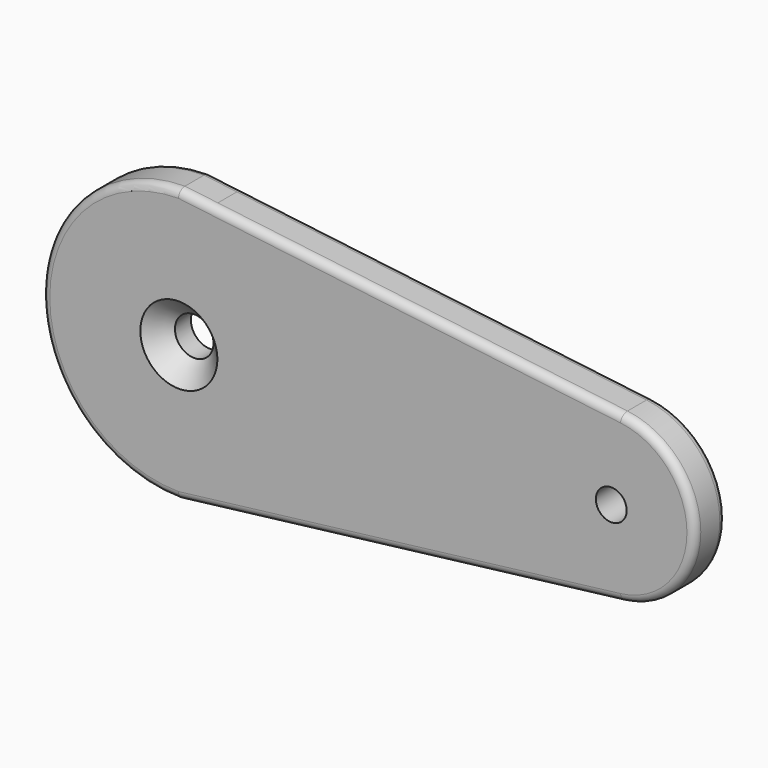
from build123d import *

# Parameters (mm, degrees)
F1_DEPTH       = 5.08
F2_T1_DEPTH    = 62.1438386925
F2_T3_DEPTH    = 62.1438386925
F2_T6_ANGLE    = 166.0840890898
F2_T8_ANGLE    = 196.1575929171
F3_T1_DEPTH    = 62.1438386925
F3_T3_DEPTH    = 62.1438386925
F3_T6_ANGLE    = 166.0840890898
F3_T8_ANGLE    = 196.1575929171
F5_D           = 5
F5_CSINK_D     = 10
F5_CSINK_ANGLE = 90
F6_D           = 4


# Not quite as in the source:
# - a fillet or chamfer that OpenCascade refuses, or shapes differently, is made with other operations: its cross-section is extruded or revolved along the edge and cut away or added


with BuildPart() as f1:
    # F0 (on Front) → F1 (new body)
    with BuildSketch(Plane.XZ):
        with BuildLine():
            Line((57.4674687515, 10.7454937358), (4.2709509748, 17.237583418))
            Line((4.2709509748, 17.237583418), (0, 17.7588092034))
            ThreePointArc((0, 17.7588092034), (-17.7588092034, 0), (0, -17.7588092034))
            Line((0, -17.7588092034), (4.2709509748, -17.237583418))
            Line((4.2709509748, -17.237583418), (57.4674687515, -10.7454937358))
            ThreePointArc((57.4674687515, -10.7454937358), (66.9813094594, 0), (57.4674687515, 10.7454937358))
        make_face()
    extrude(amount=F1_DEPTH)

    # F2: fillet of radius 1 on 4 edges, made by hand

    # F2_s2 → F2_t1 (cut)
    with BuildSketch(Plane(origin=(-6.354175572, 0, 0.7754619925), x_dir=(0, 1, 0), z_dir=(0.992635314, 0, -0.1211409647))):
        with BuildLine():
            ThreePointArc((-5.08, 16.6280211506), (-4.7871067812, 17.3351279318), (-4.08, 17.6280211506))
            Line((-4.08, 17.6280211506), (-5.08, 17.6280211506))
            Line((-5.08, 17.6280211506), (-5.08, 16.6280211506))
        make_face()
    extrude(amount=F2_T1_DEPTH, mode=Mode.SUBTRACT)

    # F2_s4 → F2_t3 (cut)
    with BuildSketch(Plane(origin=(55.3319932641, 0, 6.7527025749), x_dir=(0, 1, 0), z_dir=(-0.992635314, 0, -0.1211409647))):
        with BuildLine():
            ThreePointArc((-5.08, 16.6280211506), (-4.7871067812, 17.3351279318), (-4.08, 17.6280211506))
            Line((-4.08, 17.6280211506), (-5.08, 17.6280211506))
            Line((-5.08, 17.6280211506), (-5.08, 16.6280211506))
        make_face()
    extrude(amount=F2_T3_DEPTH, mode=Mode.SUBTRACT)

    # F2_s5 → F2_t6 (revolve, cut)
    with BuildSketch(Plane(origin=(55.3319932641, 0, 6.7527025749), x_dir=(0, 1, 0), z_dir=(-0.992635314, 0, -0.1211409647))):
        with BuildLine():
            ThreePointArc((-4.08, 17.6280211506), (-4.7871067812, 17.3351279318), (-5.08, 16.6280211506))
            Line((-5.08, 16.6280211506), (-5.08, 17.6280211506))
            Line((-5.08, 17.6280211506), (-4.08, 17.6280211506))
        make_face()
    revolve(axis=Axis((56.156091392, -5.08, 0), (0, -1, 0)), revolution_arc=F2_T6_ANGLE, mode=Mode.SUBTRACT)

    # F2_s7 → F2_t8 (revolve, cut)
    with BuildSketch(Plane(origin=(0, 0, 0), x_dir=(0, 1, 0), z_dir=(0.9900757335, 0, -0.1405348426))):
        with BuildLine():
            ThreePointArc((-5.08, 16.7588092034), (-4.7871067812, 17.4659159846), (-4.08, 17.7588092034))
            Line((-4.08, 17.7588092034), (-5.08, 17.7588092034))
            Line((-5.08, 17.7588092034), (-5.08, 16.7588092034))
        make_face()
    revolve(axis=Axis((0, -5.08, 0), (0, -1, 0)), revolution_arc=F2_T8_ANGLE, mode=Mode.SUBTRACT)

    # F3: fillet of radius 1 on 4 edges, made by hand

    # F3_s2 → F3_t1 (cut)
    with BuildSketch(Plane(origin=(55.3319932641, 0, -6.7527025749), x_dir=(0, 1, 0), z_dir=(-0.992635314, 0, 0.1211409647))):
        with BuildLine():
            ThreePointArc((0, -16.6280211506), (-0.2928932188, -17.3351279318), (-1, -17.6280211506))
            Line((-1, -17.6280211506), (0, -17.6280211506))
            Line((0, -17.6280211506), (0, -16.6280211506))
        make_face()
    extrude(amount=F3_T1_DEPTH, mode=Mode.SUBTRACT)

    # F3_s4 → F3_t3 (cut)
    with BuildSketch(Plane(origin=(-6.354175572, 0, -0.7754619925), x_dir=(0, 1, 0), z_dir=(0.992635314, 0, 0.1211409647))):
        with BuildLine():
            ThreePointArc((0, -16.6280211506), (-0.2928932188, -17.3351279318), (-1, -17.6280211506))
            Line((-1, -17.6280211506), (0, -17.6280211506))
            Line((0, -17.6280211506), (0, -16.6280211506))
        make_face()
    extrude(amount=F3_T3_DEPTH, mode=Mode.SUBTRACT)

    # F3_s5 → F3_t6 (revolve, cut)
    with BuildSketch(Plane(origin=(55.3319932641, 0, 6.7527025749), x_dir=(0, 1, 0), z_dir=(-0.992635314, 0, -0.1211409647))):
        with BuildLine():
            ThreePointArc((-1, 17.6280211506), (-0.2928932188, 17.3351279318), (0, 16.6280211506))
            Line((0, 16.6280211506), (0, 17.6280211506))
            Line((0, 17.6280211506), (-1, 17.6280211506))
        make_face()
    revolve(axis=Axis((56.156091392, 0, 0), (0, -1, 0)), revolution_arc=F3_T6_ANGLE, mode=Mode.SUBTRACT)

    # F3_s7 → F3_t8 (revolve, cut)
    with BuildSketch(Plane(origin=(0, 0, 0), x_dir=(0, 1, 0), z_dir=(0.9900757335, 0, -0.1405348426))):
        with BuildLine():
            ThreePointArc((0, 16.7588092034), (-0.2928932188, 17.4659159846), (-1, 17.7588092034))
            Line((-1, 17.7588092034), (0, 17.7588092034))
            Line((0, 17.7588092034), (0, 16.7588092034))
        make_face()
    revolve(axis=Axis((0, 0, 0), (0, -1, 0)), revolution_arc=F3_T8_ANGLE, mode=Mode.SUBTRACT)

    # F5 (through all)
    with Locations(Plane.XZ.offset(5.08)):
        with Locations((0, 0)):
            CounterSinkHole(F5_D / 2, F5_CSINK_D / 2, counter_sink_angle=F5_CSINK_ANGLE)

    # F6 (through all)
    with Locations(Plane.XZ.offset(5.08)):
        with Locations((56.156091392, 0)):
            Hole(F6_D / 2)


solid = f1.part
